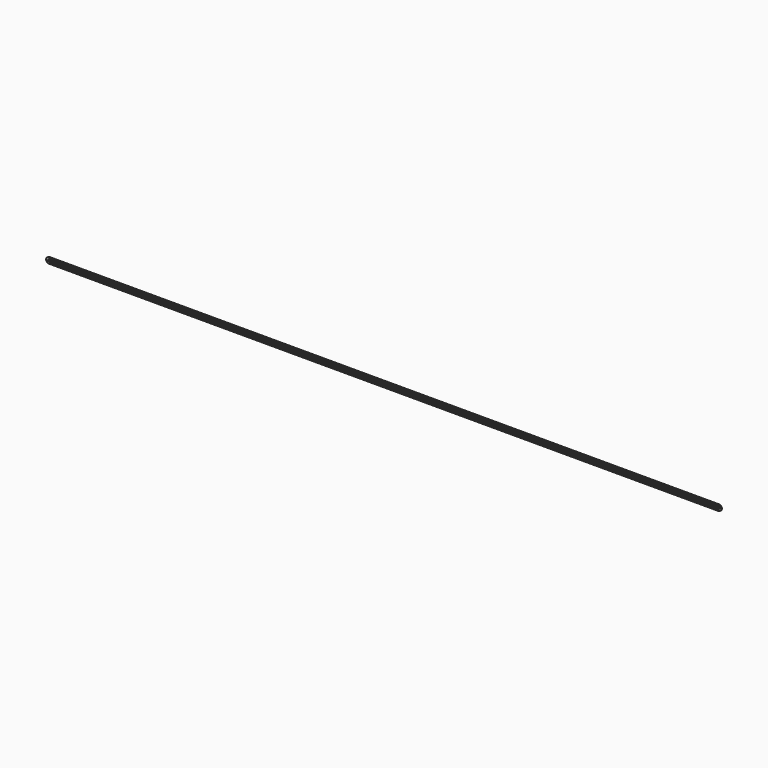
from build123d import *

# Parameters (mm, degrees)
F0_W     = 3048
F0_H     = 25.4
F1_DEPTH = 3.175
F2_R     = 12.69999
F3_R     = 4.8006
F4_DEPTH = 3.175
F5_W     = 3022.6
F5_H     = 9.6012
F6_DEPTH = 25.4


# Not quite as in the source:
# - a fillet or chamfer is up to 0.001 mm smaller than in the source, because OpenCascade refuses the exact size


with BuildPart() as f1:
    # F0 (on Front) → F1 (new body)
    with BuildSketch(Plane.XZ):
        with Locations((841.1734242707, 35.5002675663)):
            Rectangle(F0_W, F0_H)
    extrude(amount=F1_DEPTH)

    # F2 (radius 12.7 in the source; OpenCascade refuses exactly that, so slightly less here)
    f2_edges = [f1.edges().sort_by_distance(p)[0] for p in [
        (2365.173424, -1.5875, 48.200268),
        (2365.173424, -1.5875, 22.800268),
        (-682.826576, -1.5875, 48.200268),
        (-682.826576, -1.5875, 22.800268),
    ]]
    fillet(f2_edges, radius=F2_R)

    # F3 (on face) → F4 (cut)
    with BuildSketch(Plane.XZ.offset(3.175)):
        with Locations((-670.1265757293, 35.5002675663)):
            Circle(F3_R)
        with Locations((2352.4734242707, 35.5002675663)):
            Circle(F3_R)
    extrude(amount=-F4_DEPTH, mode=Mode.SUBTRACT)

    # F5 (on face) → F6 (cut)
    with BuildSketch(Plane.XZ.offset(3.175)):
        with Locations((841.1734242707, 35.5002675663)):
            Rectangle(F5_W, F5_H)
    extrude(amount=-F6_DEPTH, mode=Mode.SUBTRACT)


solid = f1.part
